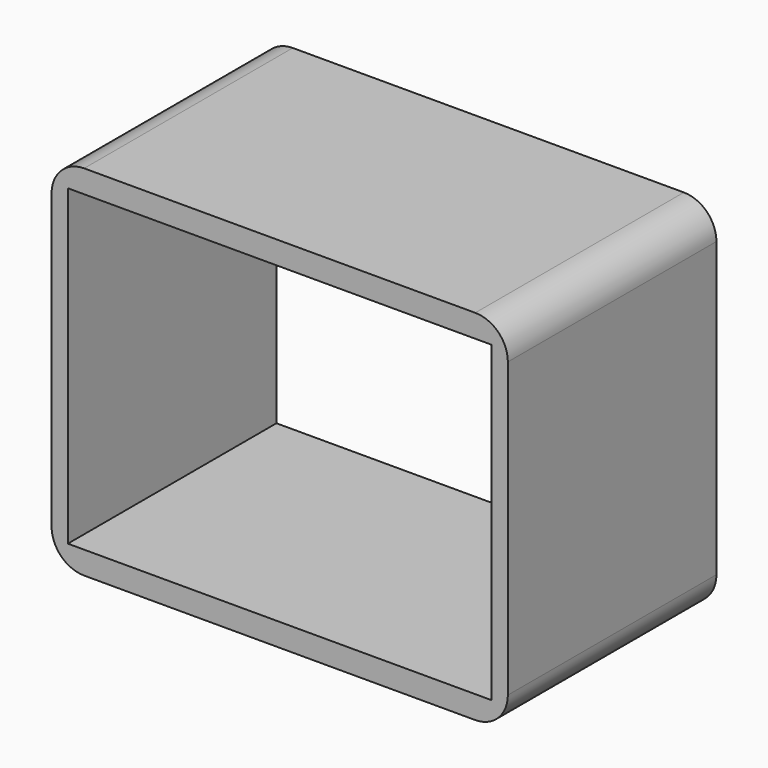
from build123d import *

# Parameters (mm, degrees)
F0_W         = 70
F0_H         = 55
F0_W_2       = 65
F0_H_2       = 48
F1_DEPTH     = 20
F2_R         = 5
F3_TEXT_SIZE = 20.1712454693
F4_DEPTH     = 1


# Not quite as in the source:
# - Text() gives the source's letters only with a copy of the font that has no kerning and outlines rounded to 1/6400 em; it was checked with that copy


with BuildPart() as f1:
    # F0 (on Front) → F1 (new body, symmetric)
    with BuildSketch(Plane.XZ):
        Rectangle(F0_W, F0_H)
        Rectangle(F0_W_2, F0_H_2, mode=Mode.SUBTRACT)
    extrude(amount=F1_DEPTH, both=True)

    # F2
    f2_edges = [f1.edges().sort_by_distance(p)[0] for p in [
        (-35, 0, -27.5),
        (35, 0, -27.5),
        (35, 0, 27.5),
        (-35, 0, 27.5),
    ]]
    fillet(f2_edges, radius=F2_R)

    # F3 (on face) → F4 (cut, symmetric)
    with BuildSketch(Plane(origin=(0, 0, -27.5), x_dir=(1, 0, 0), z_dir=(0, 0, -1))):
        with Locations((-30, -6.1168826403)):
            Text('DYMO', F3_TEXT_SIZE, font='Open Sans', text_align=(TextAlign.LEFT, TextAlign.BOTTOM))
    extrude(amount=F4_DEPTH, both=True, mode=Mode.SUBTRACT)


solid = f1.part
